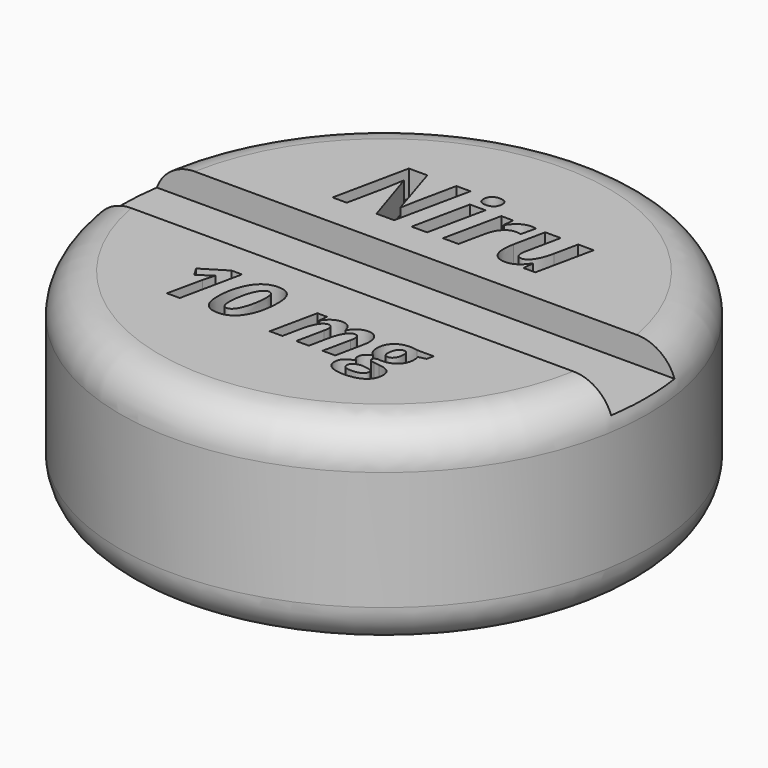
from build123d import *

# Parameters (mm, degrees)
F0_R         = 20
F1_DEPTH     = 15
F2_R         = 3
F3_W         = 40
F3_H         = 6
F4_DEPTH     = 2
F5_TEXT_SIZE = 8.0052659743
F6_DEPTH     = 2
F7_TEXT_SIZE = 6.5277777778
F8_DEPTH     = 2


# Not quite as in the source:
# - Text() gives the source's letters only with a copy of the font that has no kerning and outlines rounded to 1/6400 em; it was checked with that copy


with BuildPart() as f1:
    # F0 (on Top) → F1 (new body)
    with BuildSketch(Plane.XY):
        Circle(F0_R)
    extrude(amount=F1_DEPTH)

    # F2
    f2_edges = [f1.edges().sort_by_distance(p)[0] for p in [
        (-20, 0, 15),
        (-20, 0, 0),
    ]]
    fillet(f2_edges, radius=F2_R)

    # F3 (on face) → F4 (cut)
    with BuildSketch(Plane.XY.offset(15)):
        Rectangle(F3_W, F3_H)
    extrude(amount=-F4_DEPTH, mode=Mode.SUBTRACT)

    # F5 (on face) → F6 (cut)
    with BuildSketch(Plane.XY.offset(15)):
        with Locations((-8.5030934521, 5.5)):
            Text('Niru', F5_TEXT_SIZE, font='Open Sans', font_style=FontStyle.BOLDITALIC, text_align=(TextAlign.LEFT, TextAlign.BOTTOM))
    extrude(amount=-F6_DEPTH, mode=Mode.SUBTRACT)

    # F7 (on face) → F8 (cut)
    with BuildSketch(Plane.XY.offset(15)):
        with Locations((-9.4984266493, -10.2)):
            Text('10 mg', F7_TEXT_SIZE, font='Open Sans', font_style=FontStyle.BOLDITALIC, text_align=(TextAlign.LEFT, TextAlign.BOTTOM))
    extrude(amount=-F8_DEPTH, mode=Mode.SUBTRACT)


solid = f1.part
